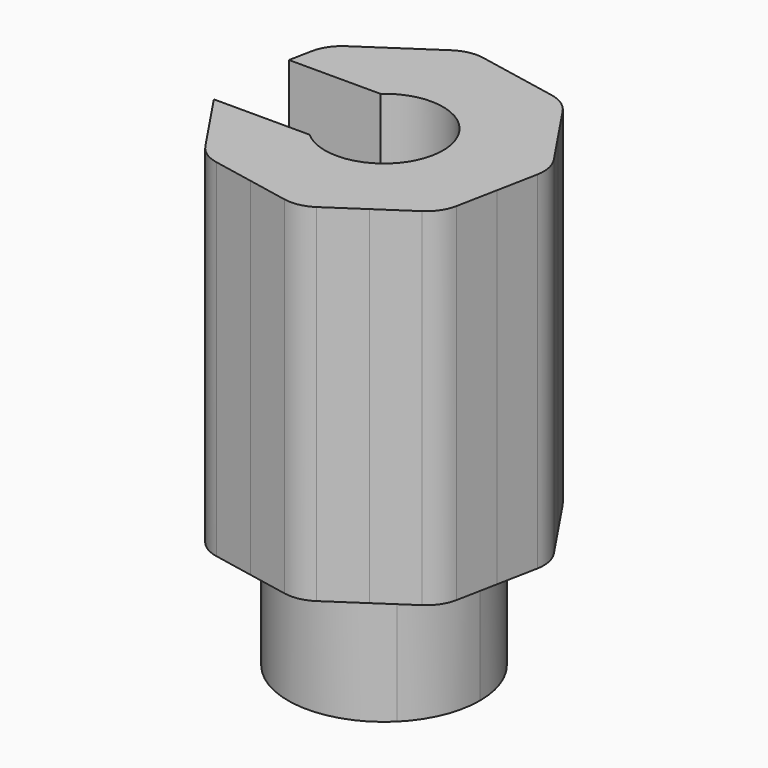
from build123d import *

# Parameters (mm, degrees)
F1_DEPTH  = 24
F2_DEPTH  = 17
F3_R      = 8
F4_DEPTH  = 40
F6_DEPTH  = 47
F8_DEPTH  = 47
F10_DEPTH = 47
F11_W     = 12
F11_H     = 90
F12_DEPTH = 25
F13_R     = 5


with BuildPart() as f1:
    # F0 (on Top) → F1 (new body)
    with BuildSketch(Plane.XY):
        with BuildLine():
            ThreePointArc((-9.1513157895, -9.2332778211), (0, -13), (9.1513157895, -9.2332778211))
            Line((9.1513157895, -9.2332778211), (-9.1513157895, -9.2332778211))
        make_face()
        with BuildLine():
            Line((-9.1513157895, -9.2332778211), (9.1513157895, -9.2332778211))
            Line((9.1513157895, -9.2332778211), (9.1513157895, 9.1513157895))
            Line((9.1513157895, 9.1513157895), (9.0700813191, 9.1513157895))
            Line((9.0700813191, 9.1513157895), (5.6315789474, 5.6820171207))
            ThreePointArc((5.6315789474, 5.6820171207), (7.3841936452, 3.0779350563), (8, 0))
            ThreePointArc((8, 0), (3.0779350563, -7.3841936452), (-5.6315789474, -5.6820171207))
            Line((-5.6315789474, -5.6820171207), (-9.1513157895, -9.2332778211))
        make_face()
        with BuildLine():
            Line((-9.1513157895, 9.0700813191), (-9.1513157895, -9.2332778211))
            Line((-9.1513157895, -9.2332778211), (-5.6315789474, -5.6820171207))
            ThreePointArc((-5.6315789474, -5.6820171207), (-7.9999204993, -0.0356651744), (-5.6820171207, 5.6315789474))
            Line((-5.6820171207, 5.6315789474), (-9.1513157895, 9.0700813191))
        make_face()
        with BuildLine():
            Line((5.6315789474, 5.6820171207), (9.0700813191, 9.1513157895))
            Line((9.0700813191, 9.1513157895), (-9.1513157895, 9.1513157895))
            Line((-9.1513157895, 9.1513157895), (-9.1513157895, 9.0700813191))
            Line((-9.1513157895, 9.0700813191), (-5.6820171207, 5.6315789474))
            ThreePointArc((-5.6820171207, 5.6315789474), (-0.0356651744, 7.9999204993), (5.6315789474, 5.6820171207))
        make_face()
        with BuildLine():
            Line((9.0700813191, 9.1513157895), (9.1513157895, 9.2332778211))
            ThreePointArc((9.1513157895, 9.2332778211), (-0.0579559084, 12.9998708114), (-9.2332778211, 9.1513157895))
            Line((-9.2332778211, 9.1513157895), (-9.1513157895, 9.0700813191))
            Line((-9.1513157895, 9.0700813191), (-9.1513157895, 9.1513157895))
            Line((-9.1513157895, 9.1513157895), (9.0700813191, 9.1513157895))
        make_face()
    extrude(amount=F1_DEPTH)

    # F0 (on Top) → F2 (join)
    with BuildSketch(Plane.XY):
        with BuildLine():
            ThreePointArc((9.1513157895, -9.2332778211), (11.9993146734, -5.0016444664), (13, 0))
            ThreePointArc((13, 0), (11.9993146734, 5.0016444664), (9.1513157895, 9.2332778211))
            Line((9.1513157895, 9.2332778211), (9.0700813191, 9.1513157895))
            Line((9.0700813191, 9.1513157895), (9.1513157895, 9.1513157895))
            Line((9.1513157895, 9.1513157895), (9.1513157895, -9.2332778211))
        make_face()
        with BuildLine():
            Line((9.0700813191, 9.1513157895), (9.1513157895, 9.2332778211))
            ThreePointArc((9.1513157895, 9.2332778211), (-0.0579559084, 12.9998708114), (-9.2332778211, 9.1513157895))
            Line((-9.2332778211, 9.1513157895), (-9.1513157895, 9.0700813191))
            Line((-9.1513157895, 9.0700813191), (-9.1513157895, 9.1513157895))
            Line((-9.1513157895, 9.1513157895), (9.0700813191, 9.1513157895))
        make_face()
        with BuildLine():
            ThreePointArc((-9.1513157895, -9.2332778211), (0, -13), (9.1513157895, -9.2332778211))
            Line((9.1513157895, -9.2332778211), (-9.1513157895, -9.2332778211))
        make_face()
        with BuildLine():
            Line((-9.1513157895, -9.2332778211), (9.1513157895, -9.2332778211))
            Line((9.1513157895, -9.2332778211), (9.1513157895, 9.1513157895))
            Line((9.1513157895, 9.1513157895), (9.0700813191, 9.1513157895))
            Line((9.0700813191, 9.1513157895), (5.6315789474, 5.6820171207))
            ThreePointArc((5.6315789474, 5.6820171207), (7.3841936452, 3.0779350563), (8, 0))
            ThreePointArc((8, 0), (3.0779350563, -7.3841936452), (-5.6315789474, -5.6820171207))
            Line((-5.6315789474, -5.6820171207), (-9.1513157895, -9.2332778211))
        make_face()
        with BuildLine():
            Line((-9.1513157895, 9.0700813191), (-9.2332778211, 9.1513157895))
            ThreePointArc((-9.2332778211, 9.1513157895), (-12.9998708114, -0.0579559084), (-9.1513157895, -9.2332778211))
            Line((-9.1513157895, -9.2332778211), (-9.1513157895, 9.0700813191))
        make_face()
        with BuildLine():
            Line((-9.1513157895, 9.0700813191), (-9.1513157895, -9.2332778211))
            Line((-9.1513157895, -9.2332778211), (-5.6315789474, -5.6820171207))
            ThreePointArc((-5.6315789474, -5.6820171207), (-7.9999204993, -0.0356651744), (-5.6820171207, 5.6315789474))
            Line((-5.6820171207, 5.6315789474), (-9.1513157895, 9.0700813191))
        make_face()
    extrude(amount=F2_DEPTH)


with BuildPart() as f4:
    # F3 (on face) → F4 (new body)
    with BuildSketch(Plane.XY.offset(24)):
        with BuildLine():
            Line((-9.1513157895, 9.0700813191), (-9.1513157895, -9.2332778211))
            ThreePointArc((-9.1513157895, -9.2332778211), (0, -13), (9.1513157895, -9.2332778211))
            Line((9.1513157895, -9.2332778211), (9.1513157895, 9.1513157895))
            Line((9.1513157895, 9.1513157895), (9.0700813191, 9.1513157895))
            Line((9.0700813191, 9.1513157895), (9.1513157895, 9.2332778211))
            ThreePointArc((9.1513157895, 9.2332778211), (-0.0337981522, 12.9421721373), (-9.1513157895, 9.0700813191))
        make_face()
        Circle(F3_R, mode=Mode.SUBTRACT)
    extrude(amount=F4_DEPTH)

    # F5 (on face) → F6 (join)
    with BuildSketch(Plane.XY.offset(17)):
        with BuildLine():
            Line((-9.1513157895, 9.0700813191), (-9.2332778211, 9.1513157895))
            ThreePointArc((-9.2332778211, 9.1513157895), (-12.9998708114, -0.0579559084), (-9.1513157895, -9.2332778211))
            Line((-9.1513157895, -9.2332778211), (-9.1513157895, 9.0700813191))
        make_face()
    extrude(amount=F6_DEPTH)

    # F7 (on face) → F8 (join)
    with BuildSketch(Plane.XY.offset(17)):
        with BuildLine():
            Line((9.0700813191, 9.1513157895), (9.1513157895, 9.1513157895))
            Line((9.1513157895, 9.1513157895), (9.1513157895, -9.2332778211))
            ThreePointArc((9.1513157895, -9.2332778211), (13, 0), (9.1513157895, 9.2332778211))
            Line((9.1513157895, 9.2332778211), (9.0700813191, 9.1513157895))
        make_face()
    extrude(amount=F8_DEPTH)

    # F9 (on face) → F10 (join)
    with BuildSketch(Plane.XY.offset(64)):
        with BuildLine():
            ThreePointArc((18.1523898541, -3.5694176815), (18.4128923896, -1.7931519315), (18.5, 0))
            ThreePointArc((18.5, 0), (17.6975039115, 5.3896526142), (15.3596372646, 10.3117187267))
            ThreePointArc((15.3596372646, 10.3117187267), (10.2443307659, 15.4046644611), (3.569417868, 18.1523898174))
            ThreePointArc((3.569417868, 18.1523898174), (-3.6489068915, 18.1365784672), (-10.3117186292, 15.3596373301))
            ThreePointArc((-10.3117186292, 15.3596373301), (-15.4046644936, 10.244330717), (-18.1523898628, 3.5694176374))
            ThreePointArc((-18.1523898628, 3.5694176374), (-18.1365784716, -3.6489068696), (-15.359637486, -10.311718397))
            ThreePointArc((-15.359637486, -10.311718397), (-10.2443309802, -15.4046643186), (-3.5694179833, -18.1523897947))
            ThreePointArc((-3.5694179833, -18.1523897947), (3.6489066832, -18.1365785091), (10.311718374, -15.3596375014))
            ThreePointArc((10.311718374, -15.3596375014), (15.4046643961, -10.2443308636), (18.1523898541, -3.5694176815))
        make_face()
        with BuildLine():
            ThreePointArc((-9.1513157895, 9.0700813191), (-0.0337981522, 12.9421721373), (9.1513157895, 9.2332778211))
            ThreePointArc((9.1513157895, 9.2332778211), (0.0579559084, -12.9998708114), (-9.2332778211, 9.1513157895))
            Line((-9.2332778211, 9.1513157895), (-9.1513157895, 9.0700813191))
        make_face(mode=Mode.SUBTRACT)
        with BuildLine():
            Line((3.949548491, -19.6308910463), (10.311718374, -15.3596375014))
            ThreePointArc((10.311718374, -15.3596375014), (3.6489066832, -18.1365785091), (-3.5694179833, -18.1523897947))
            Line((-3.5694179833, -18.1523897947), (3.949548491, -19.6308910463))
        make_face()
        with BuildLine():
            Line((-11.088383659, -16.6738887002), (-3.5694179833, -18.1523897947))
            ThreePointArc((-3.5694179833, -18.1523897947), (-10.2443309802, -15.4046643186), (-15.359637486, -10.311718397))
            Line((-15.359637486, -10.311718397), (-11.088383659, -16.6738887002))
        make_face()
        with BuildLine():
            ThreePointArc((-15.359637486, -10.311718397), (-18.1365784716, -3.6489068696), (-18.1523898628, 3.5694176374))
            Line((-18.1523898628, 3.5694176374), (-19.6308910463, -3.949548491))
            Line((-19.6308910463, -3.949548491), (-15.359637486, -10.311718397))
        make_face()
        with BuildLine():
            ThreePointArc((-18.1523898628, 3.5694176374), (-15.4046644936, 10.244330717), (-10.3117186292, 15.3596373301))
            Line((-10.3117186292, 15.3596373301), (-16.6738887002, 11.088383659))
            Line((-16.6738887002, 11.088383659), (-18.1523898628, 3.5694176374))
        make_face()
        with BuildLine():
            ThreePointArc((-10.3117186292, 15.3596373301), (-3.6489068915, 18.1365784672), (3.569417868, 18.1523898174))
            Line((3.569417868, 18.1523898174), (-3.949548491, 19.6308910463))
            Line((-3.949548491, 19.6308910463), (-10.3117186292, 15.3596373301))
        make_face()
        with BuildLine():
            ThreePointArc((3.569417868, 18.1523898174), (10.2443307659, 15.4046644611), (15.3596372646, 10.3117187267))
            Line((15.3596372646, 10.3117187267), (11.088383659, 16.6738887002))
            Line((11.088383659, 16.6738887002), (3.569417868, 18.1523898174))
        make_face()
        with BuildLine():
            ThreePointArc((15.3596372646, 10.3117187267), (17.6975039115, 5.3896526142), (18.5, 0))
            ThreePointArc((18.5, 0), (18.4128923896, -1.7931519315), (18.1523898541, -3.5694176815))
            Line((18.1523898541, -3.5694176815), (19.6308910463, 3.949548491))
            Line((19.6308910463, 3.949548491), (15.3596372646, 10.3117187267))
        make_face()
        with BuildLine():
            Line((16.6738887002, -11.088383659), (18.1523898541, -3.5694176815))
            ThreePointArc((18.1523898541, -3.5694176815), (15.4046643961, -10.2443308636), (10.311718374, -15.3596375014))
            Line((10.311718374, -15.3596375014), (16.6738887002, -11.088383659))
        make_face()
    extrude(amount=-F10_DEPTH)

    # F11 (on Right) → F12 (cut)
    with BuildSketch(Plane.YZ):
        with Locations((0, 45)):
            Rectangle(F11_W, F11_H)
    extrude(amount=-F12_DEPTH, mode=Mode.SUBTRACT)

    # F13
    f13_edges = [f4.edges().sort_by_distance(p)[0] for p in [
        (16.673889, -11.088384, 40.5),
        (3.949548, -19.630891, 40.5),
        (19.630891, 3.949548, 40.5),
        (11.088384, 16.673889, 40.5),
        (-3.949548, 19.630891, 40.5),
        (-16.673889, 11.088384, 40.5),
        (-11.088384, -16.673889, 40.5),
    ]]
    fillet(f13_edges, radius=F13_R)


solid = Compound([f1.part, f4.part])
